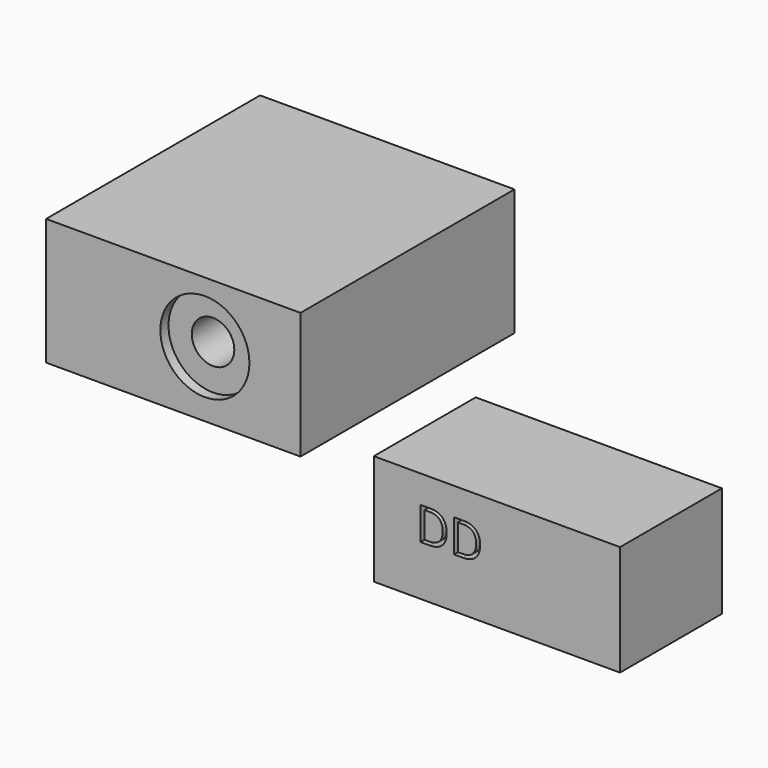
from build123d import *

# Parameters (mm, degrees)
F0_W         = 49.1057410836
F0_H         = 22.0360611565
F1_DEPTH     = 25.4
F2_TEXT_SIZE = 9.147507242
F3_DEPTH     = 12.7
F4_W         = 50.7384296507
F4_H         = 25.2387095243
F5_DEPTH     = 53.34
F6_R         = 4.2421542142
F7_DEPTH     = 53.341
F6_R_2       = 8.8810043461
F8_DEPTH     = 2.032


# Not quite as in the source:
# - Text() gives the source's letters only with a copy of the font that has no kerning and outlines rounded to 1/6400 em; it was checked with that copy


with BuildPart() as f1:
    # F0 (on Front) → F1 (new body)
    with BuildSketch(Plane.XZ):
        with Locations((-1.8508490175, 5.2522176411)):
            Rectangle(F0_W, F0_H)
    extrude(amount=F1_DEPTH)

    # F2 (on face) → F3 (cut)
    with BuildSketch(Plane.XZ.offset(25.4)):
        with Locations((-17.9714020342, 4.2201178148)):
            Text('DD', F2_TEXT_SIZE, font='Open Sans', text_align=(TextAlign.LEFT, TextAlign.BOTTOM))
    extrude(amount=-F3_DEPTH, mode=Mode.SUBTRACT)


with BuildPart() as f5:
    # F4 (on Front) → F5 (new body)
    with BuildSketch(Plane.XZ):
        with Locations((-44.0380172804, 42.6827957854)):
            Rectangle(F4_W, F4_H)
    extrude(amount=F5_DEPTH)

    # F6 (on face) → F7 (cut, through all)
    with BuildSketch(Plane.XZ.offset(53.34)):
        with Locations((-37.7394855022, 43.1757569313)):
            Circle(F6_R)
    extrude(amount=-F7_DEPTH, mode=Mode.SUBTRACT)

    # F6 (on face) → F8 (cut)
    with BuildSketch(Plane.XZ.offset(53.34)):
        with Locations((-37.7394855022, 43.1757569313)):
            Circle(F6_R_2)
        with Locations((-37.7394855022, 43.1757569313)):
            Circle(F6_R, mode=Mode.SUBTRACT)
    extrude(amount=-F8_DEPTH, mode=Mode.SUBTRACT)


solid = Compound([f1.part, f5.part])
